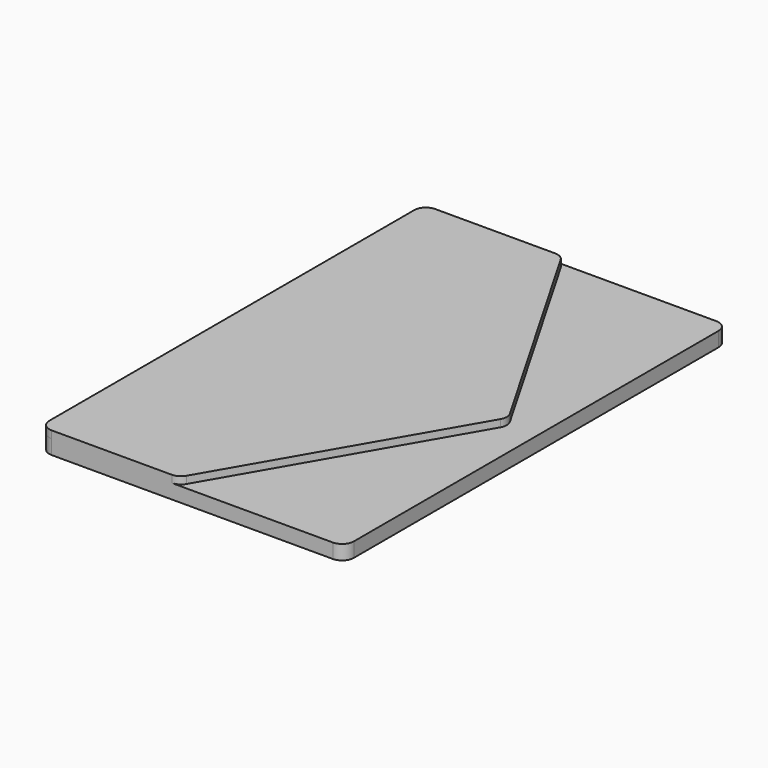
from build123d import *

# Parameters (mm, degrees)
F0_W        = 133.1540048122
F0_H        = 209.6776887774
F1_DEPTH    = 6.35
F3_R        = 5.08
F4_DEPTH    = 3.175
F5_T1_DEPTH = 10.5072040854
F5_T3_DEPTH = 28.5745000049


# Not quite as in the source:
# - a fillet or chamfer that OpenCascade refuses, or shapes differently, is made with other operations: its cross-section is extruded or revolved along the edge and cut away or added
# - two fillets or chamfers of one size are made in one step


with BuildPart() as f1:
    # F0 (on Top) → F1 (new body)
    with BuildSketch(Plane.XY):
        with Locations((0, 44.9198447168)):
            Rectangle(F0_W, F0_H)
    extrude(amount=F1_DEPTH)

    # F3
    f3_edges = [f1.edges().sort_by_distance(p)[0] for p in [
        (66.577002, -59.919, 3.175),
        (66.577002, 149.758689, 3.175),
        (-66.577002, 149.758689, 3.175),
        (-66.577002, -59.919, 3.175),
    ]]
    fillet(f3_edges, radius=F3_R)

    # F2 (on face) → F4 (join)
    with BuildSketch(Plane.XY.offset(6.35)):
        Polygon((-66.5770024061, -59.9189996719), (-6.0482673768, -59.9189996719), (54.4804676526, 44.9198447168), (-6.0482673768, 149.7586891055), (-66.5770024061, 149.7586891055), align=None)
    extrude(amount=F4_DEPTH)

    # F5: fillet of radius 5.08 on 5 edges, made by hand

    # F5_s2 → F5_t1 (cut)
    with BuildSketch(Plane.XY.offset(6.35)):
        with BuildLine():
            ThreePointArc((-8.9811490092, -59.9190996719), (-6.4411490092, -59.2385087232), (-4.581739958, -57.3790996719))
            Line((-4.581739958, -57.3790996719), (-4.493751777, -57.4298996719))
            ThreePointArc((-4.493751777, -57.4298996719), (-5.2270587876, -58.6998246719), (-5.9602791957, -59.9697996719))
            Line((-5.9602791957, -59.9697996719), (-6.0482673768, -60.0205996719))
            ThreePointArc((-6.0482673768, -60.0205996719), (-7.514708193, -60.0205996719), (-8.9811490092, -60.0206996719))
            Line((-8.9811490092, -60.0206996719), (-8.9811490092, -59.9190996719))
        make_face()
        with BuildLine():
            ThreePointArc((-8.9811490092, 149.7587891055), (-6.4411490092, 149.0781981567), (-4.581739958, 147.2187891055))
            Line((-4.581739958, 147.2187891055), (-4.493751777, 147.2695891055))
            ThreePointArc((-4.493751777, 147.2695891055), (-5.2270587876, 148.5395141055), (-5.9602791957, 149.8094891055))
            Line((-5.9602791957, 149.8094891055), (-6.0482673768, 149.8602891055))
            ThreePointArc((-6.0482673768, 149.8602891055), (-7.514708193, 149.8602891055), (-8.9811490092, 149.8603891055))
            Line((-8.9811490092, 149.8603891055), (-8.9811490092, 149.7587891055))
        make_face()
        with BuildLine():
            ThreePointArc((53.0141134389, 47.4598447168), (53.6947043877, 44.9198447168), (53.0141134389, 42.3798447168))
            Line((53.0141134389, 42.3798447168), (53.1021016199, 42.3290447168))
            ThreePointArc((53.1021016199, 42.3290447168), (53.8352354255, 43.5990697168), (54.5684558336, 44.8690447168))
            Line((54.5684558336, 44.8690447168), (54.5684558336, 44.9706447168))
            ThreePointArc((54.5684558336, 44.9706447168), (53.8352354255, 46.2406197168), (53.1021016199, 47.5106447168))
            Line((53.1021016199, 47.5106447168), (53.0141134389, 47.4598447168))
        make_face()
    extrude(amount=F5_T1_DEPTH, mode=Mode.SUBTRACT)

    # F5_s4 → F5_t3 (cut)
    with BuildSketch(Plane.XY.offset(-6.3497500025)):
        with BuildLine():
            ThreePointArc((-66.5771024061, 144.6787891055), (-65.0892048545, 148.2708915539), (-61.4971024061, 149.7587891055))
            Line((-61.4971024061, 149.7587891055), (-61.4971024061, 149.8603891055))
            ThreePointArc((-61.4971024061, 149.8603891055), (-64.0370524061, 149.8602891055), (-66.5770024061, 149.8602891055))
            Line((-66.5770024061, 149.8602891055), (-66.6786024061, 149.7586891055))
            ThreePointArc((-66.6786024061, 149.7586891055), (-66.6786024061, 147.2187391055), (-66.6787024061, 144.6787891055))
            Line((-66.6787024061, 144.6787891055), (-66.5771024061, 144.6787891055))
        make_face()
        with BuildLine():
            ThreePointArc((-66.5771024061, -54.8390996719), (-65.0892048545, -58.4312021204), (-61.4971024061, -59.9190996719))
            Line((-61.4971024061, -59.9190996719), (-61.4971024061, -60.0206996719))
            ThreePointArc((-61.4971024061, -60.0206996719), (-64.0370524061, -60.0205996719), (-66.5770024061, -60.0205996719))
            Line((-66.5770024061, -60.0205996719), (-66.6786024061, -59.9189996719))
            ThreePointArc((-66.6786024061, -59.9189996719), (-66.6786024061, -57.3790496719), (-66.6787024061, -54.8390996719))
            Line((-66.6787024061, -54.8390996719), (-66.5771024061, -54.8390996719))
        make_face()
    extrude(amount=F5_T3_DEPTH, mode=Mode.SUBTRACT)


solid = f1.part
